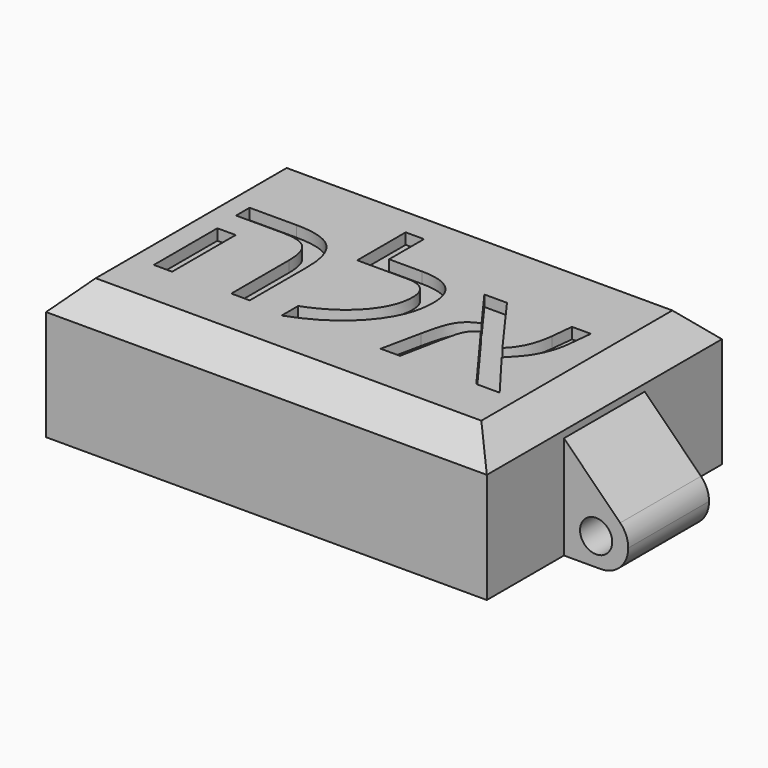
from build123d import *

# Parameters (mm, degrees)
F0_W          = 48
F0_H          = 32
F1_DEPTH      = 15
F2_W          = 44
F2_H          = 28
F3_DEPTH      = 13
F4_W          = 7
F4_H          = 11
F5_DEPTH      = 6
F6_R          = 1.75
F7_DEPTH      = 60.8
F8_T1_DEPTH   = 26
F9_W          = 44
F9_H          = 8
F10_DEPTH     = 1
F11_W         = 2
F11_H         = 10
F12_DEPTH     = 13
F13_SIZE      = 3
F14_SIZE      = 2
F16_DEPTH     = 11
F17_TEXT_SIZE = 22.2222222222
F18_DEPTH     = 1.2


# Not quite as in the source:
# - a fillet or chamfer that OpenCascade refuses, or shapes differently, is made with other operations: its cross-section is extruded or revolved along the edge and cut away or added
# - a feature names something its author has since deleted; it is built from what else it names
# - Text() gives the source's letters only with a copy of the font that has no kerning and outlines rounded to 1/6400 em; it was checked with that copy


with BuildPart() as f1:
    # F0 (on Top) → F1 (new body)
    with BuildSketch(Plane.XY):
        with Locations((24, 16)):
            Rectangle(F0_W, F0_H)
    extrude(amount=F1_DEPTH)

    # F2 (on face) → F3 (cut)
    with BuildSketch(Plane(origin=(0, 0, 0), x_dir=(1, 0, 0), z_dir=(0, 0, -1))):
        with Locations((24, -16)):
            Rectangle(F2_W, F2_H)
    extrude(amount=-F3_DEPTH, mode=Mode.SUBTRACT)

    # F4 (on face) → F5 (join)
    with BuildSketch(Plane(origin=(0, 0, 0), x_dir=(1, 0, 0), z_dir=(0, 0, -1))):
        with Locations((51.5, -16)):
            Rectangle(F4_W, F4_H)
    extrude(amount=-F5_DEPTH)

    # F6 (on face) → F7 (cut)
    with BuildSketch(Plane.XZ.offset(-10.5)):
        with Locations((51.5, 3)):
            Circle(F6_R)
    extrude(amount=-F7_DEPTH, mode=Mode.SUBTRACT)

    # F8: fillet of radius 3 on 2 edges, made by hand

    # F8_s2 → F8_t1 (cut)
    with BuildSketch(Plane.XZ.offset(-29)):
        with BuildLine():
            ThreePointArc((52, 0), (54.1213203436, 0.8786796564), (55, 3))
            Line((55, 3), (55, 0))
            Line((55, 0), (52, 0))
        make_face()
        with BuildLine():
            ThreePointArc((55, 3), (54.1213203436, 5.1213203436), (52, 6))
            Line((52, 6), (55, 6))
            Line((55, 6), (55, 3))
        make_face()
    extrude(amount=F8_T1_DEPTH, mode=Mode.SUBTRACT)

    # F9 (on face) → F10 (join)
    with BuildSketch(Plane(origin=(0, 0, 0), x_dir=(1, 0, 0), z_dir=(0, 0, -1))):
        with Locations((24, -6)):
            Rectangle(F9_W, F9_H)
    extrude(amount=-F10_DEPTH)

    # F11 (on face) → F12 (join, through all)
    with BuildSketch(Plane(origin=(0, 0, 0), x_dir=(1, 0, 0), z_dir=(0, 0, -1))):
        with Locations((25, -5)):
            Rectangle(F11_W, F11_H)
    extrude(amount=-F12_DEPTH)

    # F13
    f13_edges = [f1.edges().sort_by_distance(p)[0] for p in [
        (48, 16, 15),
        (24, 0, 15),
        (0, 16, 15),
        (24, 32, 15),
    ]]
    chamfer(f13_edges, length=F13_SIZE)

    # F14
    f14_edges = [f1.edges().sort_by_distance(p)[0] for p in [
        (24, 30, 13),
        (46, 16, 13),
        (13, 2, 13),
        (36, 2, 13),
        (2, 16, 13),
    ]]
    chamfer(f14_edges, length=F14_SIZE)

    # F15 (on face) → F16 (join, through all)
    with BuildSketch(Plane.XZ.offset(-10.5)):
        with BuildLine():
            Line((48, 11.2426406871), (48, 6))
            Line((48, 6), (52, 6))
            ThreePointArc((52, 6), (53.1480502971, 5.7716385975), (54.1213203436, 5.1213203436))
            Line((54.1213203436, 5.1213203436), (48, 11.2426406871))
        make_face()
    extrude(amount=-F16_DEPTH)

    # F17 (on face) → F18 (cut)
    with BuildSketch(Plane.XY.offset(15)):
        with Locations((3.4635416667, 8)):
            Text('הלא', F17_TEXT_SIZE, font='Arimo', text_align=(TextAlign.LEFT, TextAlign.BOTTOM))
    extrude(amount=-F18_DEPTH, mode=Mode.SUBTRACT)


solid = f1.part
